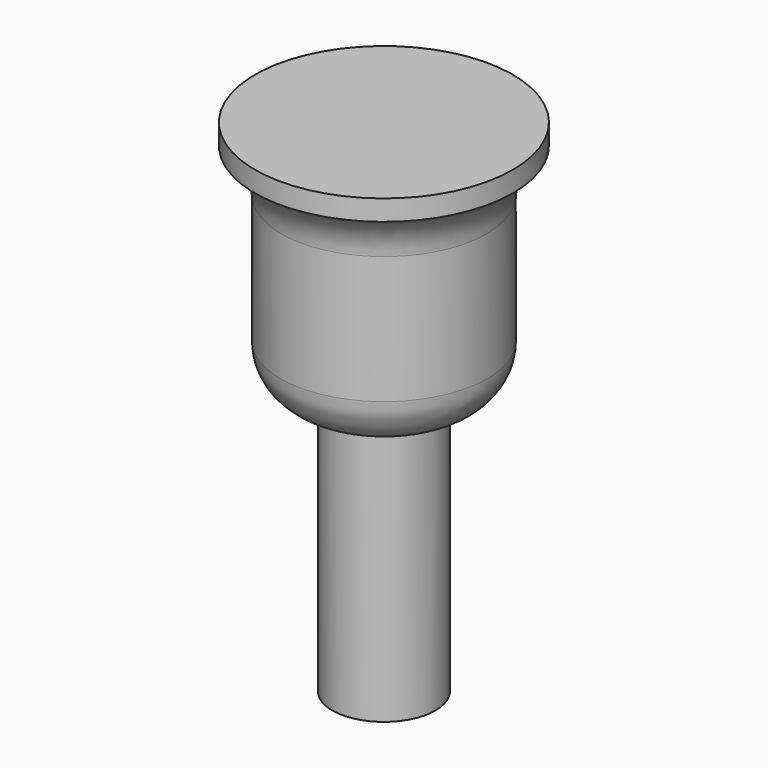
from build123d import *

# Parameters (mm, degrees)
F0_R      = 6.35
F1_DEPTH  = 19.05
F2_R      = 4.826
F3_DEPTH  = 19.051
F4_R      = 6.35
F5_DEPTH  = 12.7
F6_R      = 2.8575
F7_DEPTH  = 8.89
F8_R      = 12.7
F8_R_2    = 6.35
F9_DEPTH  = 2.032
F10_R     = 12.7
F11_DEPTH = 25.4
F12_R     = 10.795
F13_DEPTH = 25.4
F14_R     = 15.875
F15_DEPTH = 2.54


# Not quite as in the source:
# - a fillet or chamfer that OpenCascade refuses, or shapes differently, is made with other operations: its cross-section is extruded or revolved along the edge and cut away or added


with BuildPart() as f1:
    # F0 (on Top) → F1 (new body)
    with BuildSketch(Plane.XY):
        Circle(F0_R)
    extrude(amount=F1_DEPTH)

    # F2 (on face) → F3 (cut, through all)
    with BuildSketch(Plane.XY.offset(19.05)):
        Circle(F2_R)
    extrude(amount=-F3_DEPTH, mode=Mode.SUBTRACT)

    # F4 (on face) → F5 (join)
    with BuildSketch(Plane.XY.offset(19.05)):
        Circle(F4_R)
    extrude(amount=F5_DEPTH)

    # F6 (on face) → F7 (cut)
    with BuildSketch(Plane(origin=(0, 0, 19.05), x_dir=(1, 0, 0), z_dir=(0, 0, -1))):
        Circle(F6_R)
    extrude(amount=-F7_DEPTH, mode=Mode.SUBTRACT)


with BuildPart() as f9:
    # F8 (on face) → F9 (new body)
    with BuildSketch(Plane.XY.offset(31.75)):
        Circle(F8_R)
        Circle(F8_R_2, mode=Mode.SUBTRACT)
    extrude(amount=F9_DEPTH)

    # F10 (on face) → F11 (join)
    with BuildSketch(Plane.XY.offset(33.782)):
        Circle(F10_R)
    extrude(amount=F11_DEPTH)

    # F12 (on face) → F13 (cut)
    with BuildSketch(Plane.XY.offset(59.182)):
        Circle(F12_R)
    extrude(amount=-F13_DEPTH, mode=Mode.SUBTRACT)

    # F14 (on face) → F15 (join)
    with BuildSketch(Plane.XY.offset(59.182)):
        Circle(F14_R)
    extrude(amount=F15_DEPTH)

    # F16: fillet of radius 6.35 on 3 edges, made by hand

    # F16_s1 → F16_t2 (revolve)
    with BuildSketch(Plane.XZ):
        with BuildLine():
            ThreePointArc((15.8747999696, 59.1823463926), (13.5503822614, 56.8576225725), (12.6996, 53.6821811755))
            Line((12.6996, 53.6821811755), (12.0644634315, 53.6821811755))
            ThreePointArc((12.0644634315, 53.6821811755), (12.0648634315, 56.4320905877), (12.0648634315, 59.182))
            Line((12.0648634315, 59.182), (12.7, 59.8171365685))
            ThreePointArc((12.7, 59.8171365685), (14.2873999848, 59.8171365685), (15.557183398, 59.7323629143))
            Line((15.557183398, 59.7323629143), (15.8747999696, 59.1823463926))
        make_face()
    revolve(axis=Axis((0, 0, 59.182), (0, 0, 1)))

    # F16_s3 → F16_t4 (revolve, cut)
    with BuildSketch(Plane.XZ):
        with BuildLine():
            ThreePointArc((12.7004, 38.100965612), (10.8404694904, 33.6102133219), (6.3500000608, 31.7496))
            Line((6.3500000608, 31.7496), (6.3500966354, 31.1144634388))
            ThreePointArc((6.3500966354, 31.1144634388), (9.5250000304, 31.1148634315), (12.7, 31.1148634315))
            Line((12.7, 31.1148634315), (13.3351365685, 31.75))
            ThreePointArc((13.3351365685, 31.75), (13.3351365685, 34.925482806), (13.3355365685, 38.100965612))
            Line((13.3355365685, 38.100965612), (12.7004, 38.100965612))
        make_face()
    revolve(axis=Axis((0, 0, 31.75), (0, 0, 1)), mode=Mode.SUBTRACT)


solid = Compound([f1.part, f9.part])
